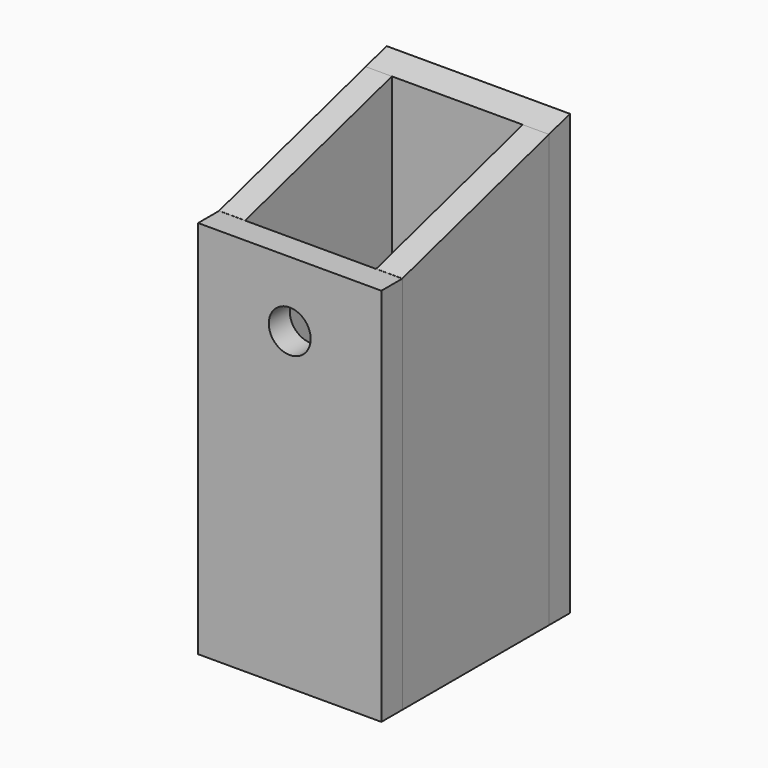
from build123d import *

# Parameters (mm, degrees)
F0_W     = 100
F0_H     = 140
F1_DEPTH = 20
F2_W     = 140
F2_H     = 289.9223208091
F2_R     = 16
F3_DEPTH = 20
F5_DEPTH = 20
F8_DEPTH = 140


with BuildPart() as f1:
    # F0 (on Top) → F1 (new body)
    with BuildSketch(Plane.XY):
        Rectangle(F0_W, F0_H)
    extrude(amount=F1_DEPTH)

    # F4 (on face) → F5 (join)
    with BuildSketch(Plane(origin=(-50, 0, 0), x_dir=(0, -1, 0), z_dir=(-1, 0, 0))):
        Polygon((-70, 330), (-70, 0), (70, 0), (70, 290), align=None)
    extrude(amount=F5_DEPTH)

    # F6: F1 across plane


with BuildPart() as f3:
    # F2 (on face) → F3 (new body)
    with BuildSketch(Plane.XZ.offset(70)):
        with Locations((0, 144.9611604046)):
            Rectangle(F2_W, F2_H)
        with Locations((0, 239.9223208091)):
            Circle(F2_R, mode=Mode.SUBTRACT)
    extrude(amount=F3_DEPTH)


with BuildPart() as f1_1:
    add(f1.part)
    add(f1.part.mirror(Plane.YZ))


with BuildPart() as f8:
    # F7 (on face) → F8 (new body)
    with BuildSketch(Plane(origin=(-70, 0, 0), x_dir=(0, -1, 0), z_dir=(-1, 0, 0))):
        Polygon((-70, 0), (-70, 330), (-90, 335.7142857143), (-90, 0), align=None)
    extrude(amount=-F8_DEPTH)


solid = Compound([f3.part, f1_1.part, f8.part])
